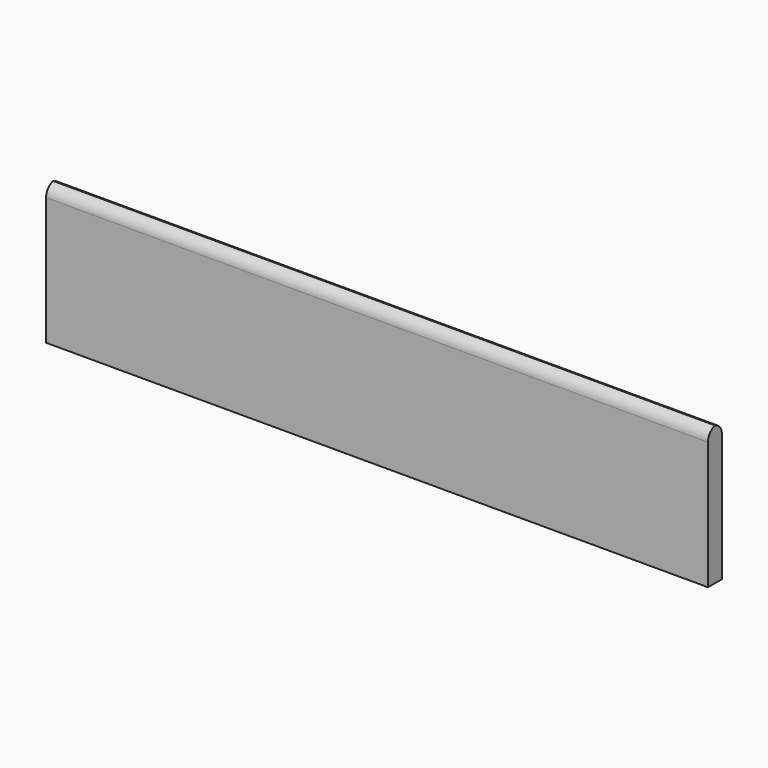
from build123d import *

# Parameters (mm, degrees)
F0_W        = 723.9
F0_H        = 152.4
F1_DEPTH    = 19.05
F2_T1_DEPTH = 787.4


# Not quite as in the source:
# - a fillet or chamfer that OpenCascade refuses, or shapes differently, is made with other operations: its cross-section is extruded or revolved along the edge and cut away or added


with BuildPart() as f1:
    # F0 (on Front) → F1 (new body)
    with BuildSketch(Plane.XZ):
        Rectangle(F0_W, F0_H)
    extrude(amount=F1_DEPTH)

    # F2: fillet of radius 12.7 on 2 edges, made by hand

    # F2_s2 → F2_t1 (cut)
    with BuildSketch(Plane.YZ.offset(-393.7)):
        with BuildLine():
            ThreePointArc((-12.7, 76.2), (-3.7197438789, 72.4802561211), (0, 63.5))
            Line((0, 63.5), (0, 76.2))
            Line((0, 76.2), (-12.7, 76.2))
        make_face()
        with BuildLine():
            ThreePointArc((-6.35, 76.2), (-15.3302561211, 72.4802561211), (-19.05, 63.5))
            Line((-19.05, 63.5), (-19.05, 76.2))
            Line((-19.05, 76.2), (-6.35, 76.2))
        make_face()
    extrude(amount=F2_T1_DEPTH, mode=Mode.SUBTRACT)


solid = f1.part
